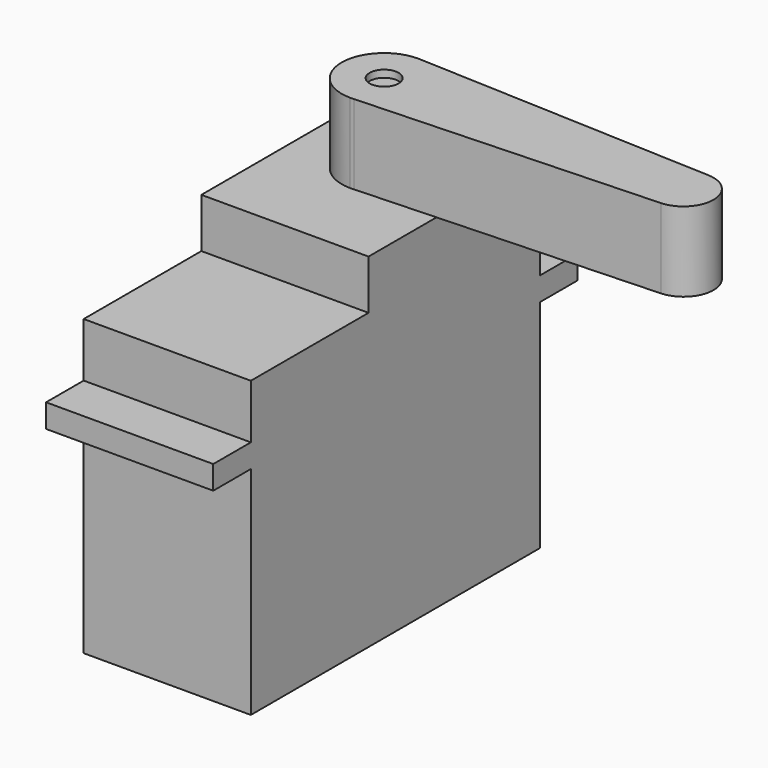
from build123d import *

# Parameters (mm, degrees)
F0_W     = 3.302
F0_H     = 1.651
F0_W_2   = 15.0622
F0_H_2   = 3.4798
F1_DEPTH = 5.87375
F2_R     = 1.016
F3_DEPTH = 5.588
F4_DEPTH = 5.08


with BuildPart() as f1:
    # F0 (on Right) → F1 (new body, symmetric)
    with BuildSketch(Plane.YZ):
        Polygon((12.7, 6.5278), (12.7, 10.3378), (-2.3622, 10.3378), (-12.7, 10.3378), (-12.7, 6.5278), (-12.7, 4.8768), (-12.7, -10.3378), (12.7, -10.3378), (12.7, 4.8768), align=None)
        with Locations((-14.351, 5.7023)):
            Rectangle(F0_W, F0_H)
        with Locations((5.1689, 12.0777)):
            Rectangle(F0_W_2, F0_H_2)
        with Locations((14.351, 5.7023)):
            Rectangle(F0_W, F0_H)
    extrude(amount=F1_DEPTH, both=True)

    # F2 (on face) → F4 (join)
    with BuildSketch(Plane.XY.offset(13.8176)):
        with Locations((0, 6.35)):
            Circle(F2_R)
    extrude(amount=F4_DEPTH)


with BuildPart() as f3:
    # F2 (on face) → F3 (new body)
    with BuildSketch(Plane.XY.offset(13.8176)):
        with BuildLine():
            Line((21.1262666217, 8.4563812185), (0, 9.3345))
            ThreePointArc((0, 9.3345), (-2.9845, 6.35), (0, 3.3655))
            Line((0, 3.3655), (0.2476751405, 3.3757946818))
            Line((0.2476751405, 3.3757946818), (21.1262666217, 4.2436187815))
            ThreePointArc((21.1262666217, 4.2436187815), (23.146914337, 6.35), (21.1262666217, 8.4563812185))
        make_face()
        with Locations((0, 6.35)):
            Circle(F2_R, mode=Mode.SUBTRACT)
        with BuildLine():
            Line((0.2476751405, 3.3757946818), (0, 3.3655))
            ThreePointArc((0, 3.3655), (0.1239444994, 3.3680747811), (0.2476751405, 3.3757946818))
        make_face()
    extrude(amount=F3_DEPTH)


solid = Compound([f1.part, f3.part])
